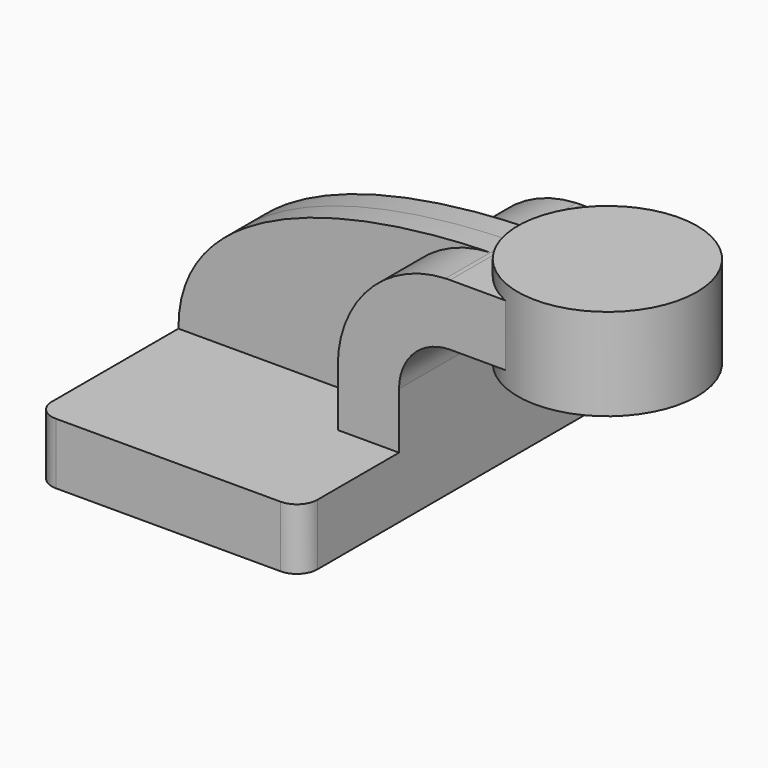
from build123d import *

# Parameters (mm, degrees)
F1_DEPTH = 63.5
F2_DEPTH = 25.4
F3_DEPTH = 7.9375
F5_R     = 6.35


# Not quite as in the source:
# - a feature names something its author has since deleted; it is built from what else it names


with BuildPart() as f1:
    # F0 (on Front) → F1 (new body, symmetric)
    with BuildSketch(Plane.XZ):
        Polygon((24.9004629219, 11.984025088), (-38.5995370781, 11.984025088), (-38.5995370781, -7.065974912), (43.9504629219, -7.065974912), (43.9504629219, 11.984025088), align=None)
    extrude(amount=F1_DEPTH, both=True)

    # F0 (on Front) → F2 (join, symmetric)
    with BuildSketch(Plane.XZ):
        with BuildLine():
            Line((24.9004629219, 29.459225088), (24.9004629219, 11.984025088))
            Line((24.9004629219, 11.984025088), (43.9504629219, 11.984025088))
            Line((43.9504629219, 11.984025088), (43.9504629219, 29.459225088))
            ThreePointArc((43.9504629219, 29.459225088), (48.6001427706, 40.6845452393), (59.8254629219, 45.334225088))
            Line((59.8254629219, 45.334225088), (65.5219778419, 45.334225088))
            Line((65.5219778419, 45.334225088), (88.4004629219, 45.334225088))
            Line((88.4004629219, 45.334225088), (88.4004629219, 64.384225088))
            Line((88.4004629219, 64.384225088), (65.4512095848, 64.384225088))
            Line((65.4512095848, 64.384225088), (59.8254629219, 64.384225088))
            add(Edge.make_bspline(
                [(58.4085351023, 64.3554704527), (58.8803787931, 64.3662992509), (59.3526984445, 64.3758829837), (59.8254629219, 64.384225088)],
                knots=[110.4908750185, 110.4908750185, 110.4908750185, 110.4908750185, 111.5045361635, 111.5045361635, 111.5045361635, 111.5045361635], degree=3))
            ThreePointArc((58.4085351023, 64.3554704527), (34.6337794817, 53.6487829684), (24.9004629219, 29.459225088))
        make_face()
    extrude(amount=F2_DEPTH, both=True)

    # F0 (on Front) → F3 (join, symmetric)
    with BuildSketch(Plane.XZ):
        with BuildLine():
            add(Edge.make_bspline(
                [(-38.5995370781, 11.984025088), (-38.8000023371, 47.2016469024), (6.976730171, 63.1751121082), (58.4085351023, 64.3554704527)],
                knots=[0, 0, 0, 0, 110.4908750185, 110.4908750185, 110.4908750185, 110.4908750185], degree=3))
            Line((-38.5995370781, 11.984025088), (24.9004629219, 11.984025088))
            Line((24.9004629219, 11.984025088), (24.9004629219, 29.459225088))
            ThreePointArc((24.9004629219, 29.459225088), (34.6337794817, 53.6487829684), (58.4085351023, 64.3554704527))
        make_face()
    extrude(amount=F3_DEPTH, both=True)

    # F0 (on Front) → F4 (revolve)
    with BuildSketch(Plane.XZ):
        Polygon((88.4004629219, 69.134025088), (88.4004629219, 64.384225088), (88.4004629219, 45.334225088), (88.4004629219, 40.559025088), (116.2512095848, 40.559025088), (116.2512095848, 69.134025088), align=None)
    revolve(axis=Axis((88.4004629219, 0, 54.846525088), (0, 0, -1)))

    # F5
    f5_edges = [f1.edges().sort_by_distance(p)[0] for p in [
        (-38.599537, -63.5, 2.459025),
        (43.950463, -63.5, 2.459025),
        (-38.599537, 63.5, 2.459025),
        (43.950463, 63.5, 2.459025),
    ]]
    fillet(f5_edges, radius=F5_R)


solid = f1.part
